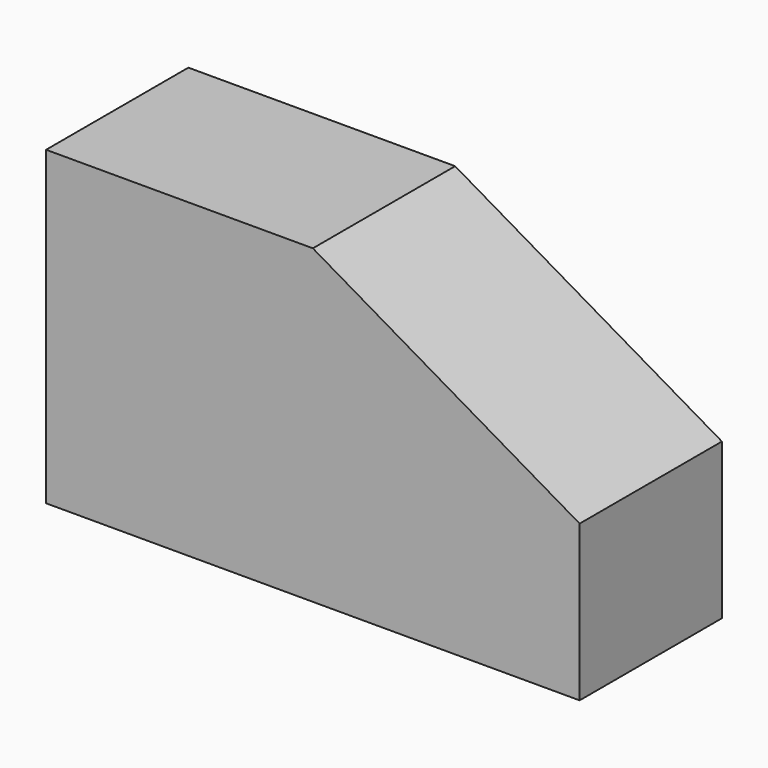
from build123d import *

# Parameters (mm, degrees)
F0_W     = 60
F0_H     = 35
F1_DEPTH = 20
F3_DEPTH = 25


# Not quite as in the source:
# - a feature names something its author has since deleted; it is built from what else it names


with BuildPart() as f1:
    # F0 (on Front) → F1 (new body)
    with BuildSketch(Plane.XZ):
        with Locations((30, 17.5)):
            Rectangle(F0_W, F0_H)
    extrude(amount=F1_DEPTH)

    # F2 (on face) → F3 (cut)
    with BuildSketch(Plane.XZ.offset(20)):
        Polygon((60, 35), (30, 35), (60, 17.5), align=None)
    extrude(amount=-F3_DEPTH, mode=Mode.SUBTRACT)


solid = f1.part
